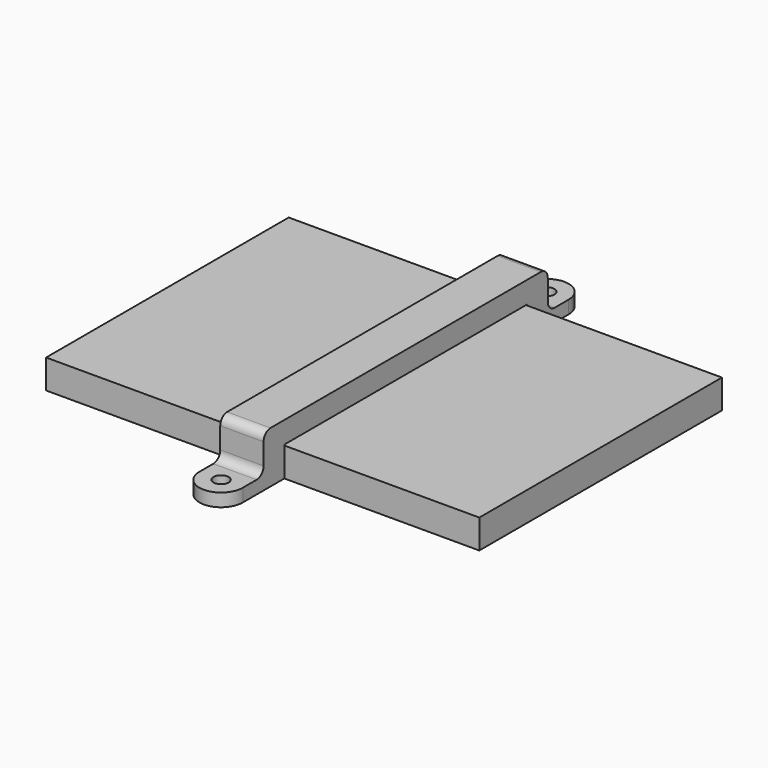
from build123d import *

# Parameters (mm, degrees)
F0_W     = 100
F0_H     = 70
F1_DEPTH = 6.7
F2_R     = 1.75
F3_DEPTH = 3
F2_W     = 10
F2_H     = 6
F4_DEPTH = 6.9
F5_W     = 10
F5_H     = 82
F6_DEPTH = 5
F7_R     = 2


with BuildPart() as f1:
    # F0 (on Top) → F1 (new body)
    with BuildSketch(Plane.XY):
        Rectangle(F0_W, F0_H)
    extrude(amount=F1_DEPTH)


with BuildPart() as f3:
    # F2 (on Top) → F3 (new body)
    with BuildSketch(Plane.XY):
        with BuildLine():
            ThreePointArc((-5, 47), (0, 42), (5, 47))
            ThreePointArc((5, 47), (0, 52), (-5, 47))
        make_face()
        with Locations((0, 47)):
            Circle(F2_R, mode=Mode.SUBTRACT)
        with BuildLine():
            Line((5, 41), (5, 47))
            ThreePointArc((5, 47), (0, 42), (-5, 47))
            Line((-5, 47), (-5, 41))
            Line((-5, 41), (5, 41))
        make_face()
    extrude(amount=F3_DEPTH)

    # F2 (on Top) → F4 (join)
    with BuildSketch(Plane.XY):
        with Locations((0, 38)):
            Rectangle(F2_W, F2_H)
    extrude(amount=F4_DEPTH)



with BuildPart() as f3b:
    # F2 (on Top) → F3, piece 2 (new body)
    with BuildSketch(Plane.XY):
        with BuildLine():
            ThreePointArc((-5, -47), (0, -52), (5, -47))
            ThreePointArc((5, -47), (0, -42), (-5, -47))
        make_face()
        with Locations((0, -47)):
            Circle(F2_R, mode=Mode.SUBTRACT)
        with BuildLine():
            ThreePointArc((-5, -47), (0, -42), (5, -47))
            Line((5, -47), (5, -41))
            Line((5, -41), (-5, -41))
            Line((-5, -41), (-5, -47))
        make_face()
    extrude(amount=F3_DEPTH)

    # F2 (on Top) → F4, piece 2 (join)
    with BuildSketch(Plane.XY):
        with Locations((0, -38)):
            Rectangle(F2_W, F2_H)
    extrude(amount=F4_DEPTH)


with BuildPart() as f3_1:
    add(f3.part)

    add(f3b.part)  # F6 merges F3b
    # F5 (on face) → F6 (join)
    with BuildSketch(Plane.XY.offset(6.9)):
        Rectangle(F5_W, F5_H)
    extrude(amount=F6_DEPTH)

    # F7
    f7_edges = [f3_1.edges().sort_by_distance(p)[0] for p in [
        (0, 41, 11.9),
        (0, -41, 11.9),
        (0, -41, 3),
        (0, 41, 3),
    ]]
    fillet(f7_edges, radius=F7_R)


solid = Compound([f1.part, f3_1.part])
